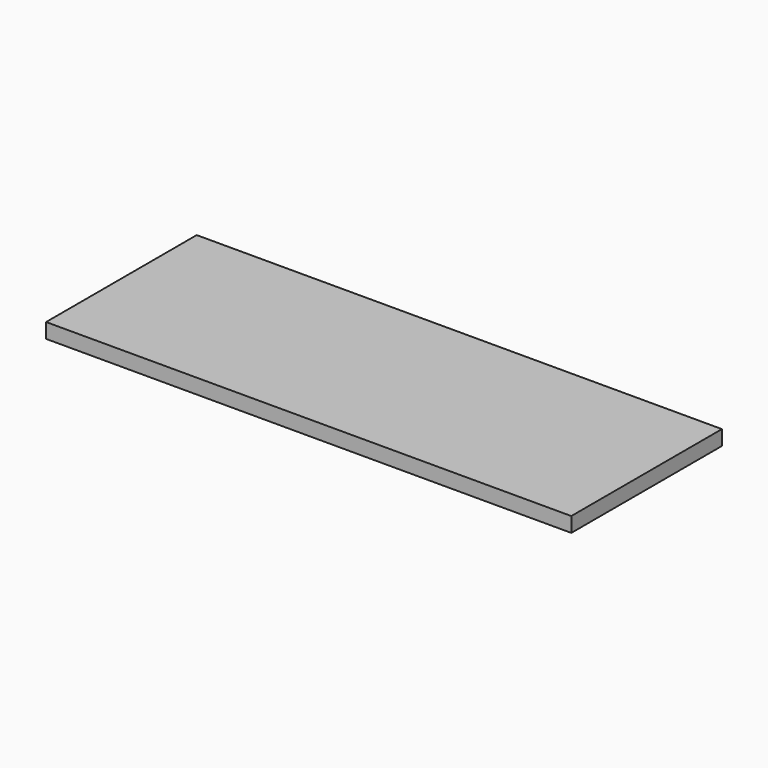
from build123d import *

# Parameters (mm, degrees)
F0_W     = 673.1
F0_H     = 241.3
F1_DEPTH = 19.05


# Not quite as in the source:
# - a length typed as a fraction of an inch, garbled in the dataset ("3 / 203.2 mm" for 3/8 in), is restored


with BuildPart() as f1:
    # F0 (on Top) → F1 (new body)
    with BuildSketch(Plane.XY):
        Rectangle(F0_W, F0_H)
    extrude(amount=F1_DEPTH)


solid = f1.part
